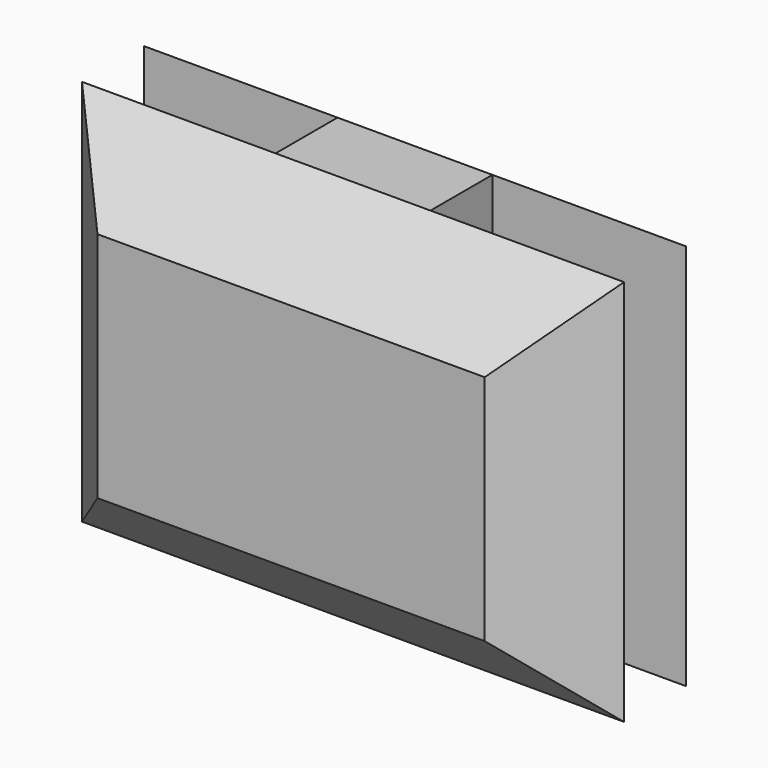
from build123d import *

# Parameters (mm, degrees)
F0_W     = 4
F0_H     = 2
F1_DEPTH = 10
F2_SIZE  = 1.99999
F3_SIZE  = 1.99999


# Not quite as in the source:
# - a fillet or chamfer is up to 0.001 mm smaller than in the source, because OpenCascade refuses the exact size


with BuildPart() as f1:
    # F0 (on Top) → F1 (new body)
    with BuildSketch(Plane.XY):
        Polygon((-7, 3), (-7, 1), (-2, 1), (2, 1), (7, 1), (7, 3), align=None)
        Rectangle(F0_W, F0_H)
        Polygon((-2, -1), (-7, -1), (-7, -3), (7, -3), (7, -1), (2, -1), align=None)
    extrude(amount=F1_DEPTH)

    # F2 (size 2 in the source; OpenCascade refuses exactly that, so slightly less here)
    f2_edges = [f1.edges().sort_by_distance(p)[0] for p in [
        (-7, 3, 5),
        (7, 3, 5),
        (7, -3, 5),
        (-7, -3, 5),
    ]]
    chamfer(f2_edges, length=F2_SIZE)

    # F3 (size 2 in the source; OpenCascade refuses exactly that, so slightly less here)
    f3_edges = [f1.edges().sort_by_distance(p)[0] for p in [
        (0, 3, 10),
        (0, -3, 10),
        (0, -3, 0),
        (0, 3, 0),
    ]]
    chamfer(f3_edges, length=F3_SIZE)


solid = f1.part
